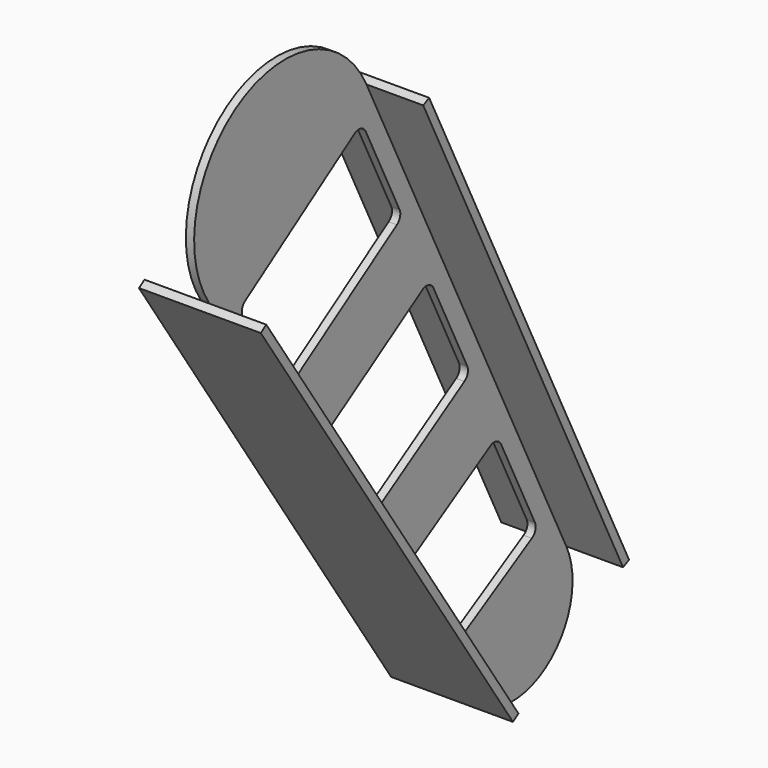
from build123d import *

# Parameters (mm, degrees)
F2_DEPTH = 11.1125
F3_W     = 76.2
F3_H     = 760.3047809925
F3_W_2   = 11.1125
F4_DEPTH = 11.1125
F5_W     = 76.2
F5_H     = 760.3047809925
F5_W_2   = 11.1125
F6_DEPTH = 11.1125


# Not quite as in the source:
# - a length typed as a fraction of an inch, garbled in the dataset ("3 / 203.2 mm" for 3/8 in), is restored


with BuildPart() as f2:
    # F1 (on face) → F2 (new body)
    with BuildSketch(Plane.YZ):
        with BuildLine():
            Line((91.1791006611, 248.0211066645), (-244.2313490084, 930.3430176805))
            ThreePointArc((-244.2313490084, 930.3430176805), (-457.2, 995.0936292205), (-507.6086509916, 778.282061482))
            Line((-507.6086509916, 778.2820614821), (-84.4057673278, 146.6471358655))
            ThreePointArc((-84.4057673278, 146.6471358655), (50.8, 115.2118189755), (91.1791006611, 248.0211066645))
        make_face()
        with BuildLine():
            ThreePointArc((-171.1045716164, 321.6783965077), (-172.951087632, 331.5040451939), (-167.114914439, 339.6214386156))
            Line((-167.114914439, 339.6214386156), (-36.3148932715, 418.5429465727))
            ThreePointArc((-36.3148932715, 418.5429465727), (-26.1769388687, 419.8548999412), (-18.3564419502, 413.2716508147))
            Line((-18.3564419502, 413.2716508147), (38.4369639182, 297.7374291963))
            ThreePointArc((38.4369639182, 297.7374291963), (39.1903819803, 288.4404814306), (33.3895763356, 281.1362682351))
            Line((33.3895763356, 281.1362682351), (-84.1895763356, 213.2519127894))
            ThreePointArc((-84.1895763356, 213.2519127894), (-93.4156133399, 211.8803743364), (-101.0902972515, 217.1813274006))
            Line((-101.0902972515, 217.1813274006), (-171.1045716164, 321.6783965077))
        make_face(mode=Mode.SUBTRACT)
        with BuildLine():
            ThreePointArc((-311.133120346, 530.6725347217), (-313.0170671845, 540.3240907704), (-307.4457804185, 548.4273341718))
            Line((-307.4457804185, 548.4273341718), (-150.2040222582, 649.4231471517))
            ThreePointArc((-150.2040222582, 649.4231471517), (-139.9349605516, 650.9722969045), (-131.9432536871, 644.3400940516))
            Line((-131.9432536871, 644.3400940516), (-75.1498478186, 528.8058724331))
            ThreePointArc((-75.1498478186, 528.8058724331), (-74.3341151725, 519.7204630371), (-79.8191746138, 512.4318275976))
            Line((-79.8191746138, 512.4318275976), (-223.8400642778, 422.4731671291))
            ThreePointArc((-223.8400642778, 422.4731671291), (-233.2289400031, 420.8264391554), (-241.1188459812, 426.1754656147))
            Line((-241.1188459812, 426.1754656147), (-311.133120346, 530.6725347217))
        make_face(mode=Mode.SUBTRACT)
        with BuildLine():
            ThreePointArc((-451.1616690757, 739.6666729358), (-453.0700486814, 749.1976530431), (-447.6800561765, 757.2865018686))
            Line((-447.6800561765, 757.2865018686), (-263.9965610234, 880.3566198713))
            ThreePointArc((-263.9965610234, 880.3566198713), (-253.6404511337, 882.0731569492), (-245.5300654239, 875.4085372884))
            Line((-245.5300654239, 875.4085372884), (-188.7366595555, 759.87431567))
            ThreePointArc((-188.7366595555, 759.87431567), (-187.8814953559, 750.930274215), (-193.1588501861, 743.6586368923))
            Line((-193.1588501861, 743.6586368923), (-363.6214768428, 631.6256714009))
            ThreePointArc((-363.6214768428, 631.6256714009), (-373.1138065223, 629.7906580687), (-381.1473947108, 635.1696038288))
            Line((-381.1473947108, 635.1696038288), (-451.1616690757, 739.6666729358))
        make_face(mode=Mode.SUBTRACT)
    extrude(amount=F2_DEPTH)

    # F3 (on face) → F4 (join)
    with BuildSketch(Plane(origin=(0, 171.626899801, 84.3670043542), x_dir=(-1, 0, 0), z_dir=(0, 0.8974320931, 0.4411526247))):
        with Locations((-49.2125, 562.5105918184)):
            Rectangle(F3_W, F3_H)
        with Locations((38.1, 562.5105918184)):
            Rectangle(F3_W, F3_H)
        with Locations((-5.55625, 562.5105918184)):
            Rectangle(F3_W_2, F3_H)
    extrude(amount=F4_DEPTH)

    # F5 (on face) → F6 (join)
    with BuildSketch(Plane(origin=(0, 9.558561252, 6.404349287), x_dir=(1, 0, 0), z_dir=(0, -0.8307654265, -0.5566226785))):
        with Locations((-38.1, 548.9639251518)):
            Rectangle(F5_W, F5_H)
        with Locations((49.2125, 548.9639251518)):
            Rectangle(F5_W, F5_H)
        with Locations((5.55625, 548.9639251518)):
            Rectangle(F5_W_2, F5_H)
    extrude(amount=F6_DEPTH)


solid = f2.part
